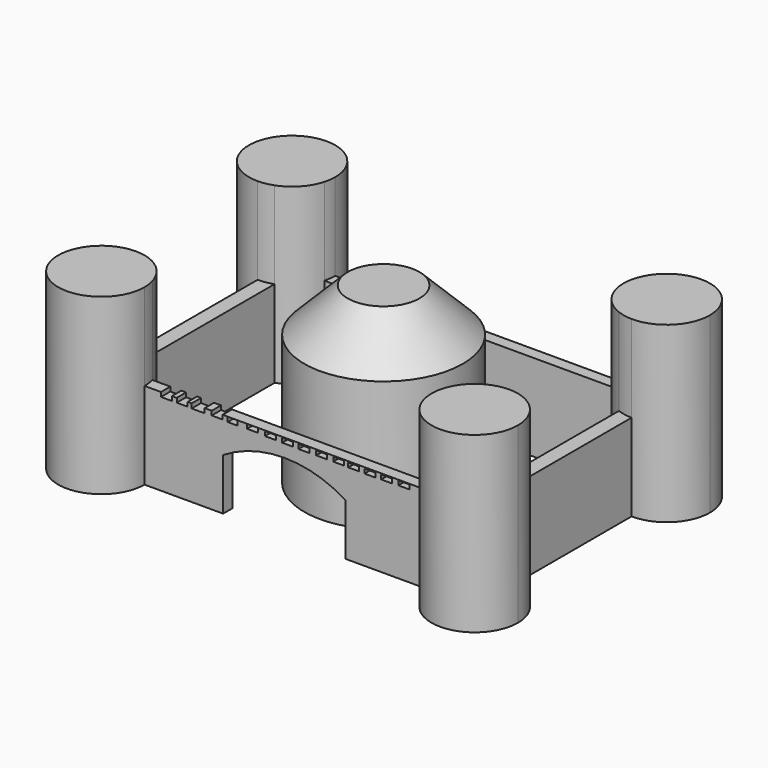
from build123d import *

# Parameters (mm, degrees)
F1_DEPTH   = 25.4
F2_DEPTH   = 50.8
F0_R       = 23.1689364428
F4_DEPTH   = 14.986
F5_W       = 3.2030940056
F5_H       = 1.273414427
F5_H_2     = 1.2491918117
F5_W_2     = 3.7871245295
F5_H_3     = 1.3221087813
F5_H_4     = 1.2197750568
F5_W_3     = 2.9007913545
F5_H_5     = 1.361253047
F1_FACE1_W = 85.1300132265
F1_FACE1_H = 25.4
F1_FACE2_W = 84.1618746061
F1_FACE2_H = 25.4
F6_DEPTH   = 7.112
F7_SIZE    = 12.7


with BuildPart() as f1:
    # F0 (on Top) → F1 (new body)
    with BuildSketch(Plane.XY):
        with BuildLine():
            Line((42.1713891774, 34.8335728049), (-41.9904854287, 34.8335728049))
            ThreePointArc((-41.9904854287, 34.8335728049), (-42.1083213465, 33.1132780775), (-42.4596279258, 31.4251184464))
            Line((-42.4596279258, 31.4251184464), (42.6703853007, 31.4251184464))
            ThreePointArc((42.6703853007, 31.4251184464), (42.3040081413, 33.1122345804), (42.1713891774, 34.8335728049))
        make_face()
    extrude(amount=F1_DEPTH)


with BuildPart() as f1b:
    # F0 (on Top) → F1, piece 2 (new body)
    with BuildSketch(Plane.XY):
        with BuildLine():
            Line((-54.6067543328, 22.2173039008), (-54.6067543328, -22.2160224009))
            ThreePointArc((-54.6067543328, -22.2160224009), (-52.3921133094, -22.4119345582), (-50.2462573349, -22.9935861489))
            Line((-50.2462573349, -22.9935861489), (-50.2462573349, 22.9948099053))
            ThreePointArc((-50.2462573349, 22.9948099053), (-52.3921183776, 22.4132012868), (-54.6067543328, 22.2173039008))
        make_face()
    extrude(amount=F1_DEPTH)


with BuildPart() as f1c:
    # F0 (on Top) → F1, piece 3 (new body)
    with BuildSketch(Plane.XY):
        with BuildLine():
            Line((-41.9913647822, -34.8335728049), (41.9646467417, -34.8335728049))
            ThreePointArc((41.9646467417, -34.8335728049), (42.0972657056, -33.1122345804), (42.463642865, -31.4251184464))
            Line((42.463642865, -31.4251184464), (-42.4599349352, -31.4251184464))
            ThreePointArc((-42.4599349352, -31.4251184464), (-42.1090561661, -33.112226656), (-41.9913645972, -34.8314121366))
            ThreePointArc((-41.9913645972, -34.8314121366), (-41.9913646434, -34.8324924707), (-41.9913647822, -34.8335728049))
        make_face()
    extrude(amount=F1_DEPTH)

    # F3 (on face) → F4 (cut)
    with BuildSketch(Plane.XZ.offset(34.8335728049)):
        with BuildLine():
            Line((-19.0204642713, 15.0923253968), (-19.0204642713, 0))
            Line((-19.0204642713, 0), (16.7462807149, 0))
            Line((16.7462807149, 0), (16.7462807149, 15.0923253968))
            ThreePointArc((16.7462807149, 15.0923253968), (-1.1370917782, 20.2000644219), (-19.0204642713, 15.0923253968))
        make_face()
    extrude(amount=-F4_DEPTH, mode=Mode.SUBTRACT)

    # F5 (on face) + F1_face1 (on face) + F1_face2 (on face) → F6 (cut)
    with BuildSketch(Plane.XZ.offset(34.8335728049)):
        with Locations((-35.5779528618, 24.7632927865)):
            Rectangle(F5_W, F5_H)
        with Locations((-30.9700351208, 24.7754040942)):
            Rectangle(F5_W, F5_H_2)
        with Locations((-26.3112029061, 24.7389456093)):
            Rectangle(F5_W_2, F5_H_3)
        with Locations((-20.7560434937, 24.7901124716)):
            Rectangle(F5_W, F5_H_4)
        with Locations((-16.2332779728, 24.6905572712)):
            Rectangle(F5_W_3, F5_H_5)
        with Locations((-10.4287816212, 24.747133255)):
            Rectangle(F5_W, F5_H)
        with Locations((-5.2050889935, 24.5689451694)):
            Rectangle(F5_W, F5_H)
        with Locations((-0.1880034979, 24.4990028441)):
            Rectangle(F5_W, F5_H)
        with Locations((4.6075105201, 24.4370289147)):
            Rectangle(F5_W, F5_H)
        with Locations((9.7847376019, 24.4842600077)):
            Rectangle(F5_W, F5_H)
        with Locations((14.7634353489, 24.4842600077)):
            Rectangle(F5_W, F5_H)
        with Locations((19.1444754601, 24.4370233268)):
            Rectangle(F5_W, F5_H)
        with Locations((23.9080954343, 24.3755578995)):
            Rectangle(F5_W, F5_H)
        with Locations((28.7535134703, 24.4615059346)):
            Rectangle(F5_W, F5_H)
        with Locations((33.7848700583, 24.5699640363)):
            Rectangle(F5_W, F5_H)
    with BuildSketch(Plane(origin=(0.1053786874, 31.4251184464, 12.7), x_dir=(1, 0, 0), z_dir=(0, -1, 0))):
        Rectangle(F1_FACE1_W, F1_FACE1_H)
    with BuildSketch(Plane(origin=(0.0904518744, 34.8335728049, 12.7), x_dir=(-1, 0, 0), z_dir=(0, 1, 0))):
        Rectangle(F1_FACE2_W, F1_FACE2_H)
    extrude(amount=-F6_DEPTH, dir=(0, -1, 0), mode=Mode.SUBTRACT)


with BuildPart() as f1d:
    # F0 (on Top) → F1, piece 4 (new body)
    with BuildSketch(Plane.XY):
        with BuildLine():
            Line((50.2462573349, 23.1690441136), (50.2462573349, -23.0913582413))
            ThreePointArc((50.2462573349, -23.0913582413), (52.3925594701, -22.5146622382), (54.6067543328, -22.3235281341))
            Line((54.6067543328, -22.3235281341), (54.6067543328, 22.3247913991))
            ThreePointArc((54.6067543328, 22.3247913991), (52.3890618107, 22.553522405), (50.2462573349, 23.1690441136))
        make_face()
    extrude(amount=F1_DEPTH)


with BuildPart() as f2:
    # F0 (on Top) → F2 (new body)
    with BuildSketch(Plane.XY):
        with BuildLine():
            ThreePointArc((-41.9904854287, 34.8335728049), (-63.5278036282, 43.7546221003), (-54.6067543328, 22.2173039008))
            ThreePointArc((-54.6067543328, 22.2173039008), (-52.3921183776, 22.4132012868), (-50.2462573349, 22.9948099053))
            ThreePointArc((-50.2462573349, 22.9948099053), (-45.3389102932, 26.2733562237), (-42.4596279258, 31.4251184464))
            ThreePointArc((-42.4596279258, 31.4251184464), (-42.1083213465, 33.1132780775), (-41.9904854287, 34.8335728049))
        make_face()
    extrude(amount=F2_DEPTH)


with BuildPart() as f2b:
    # F0 (on Top) → F2, piece 2 (new body)
    with BuildSketch(Plane.XY):
        with BuildLine():
            ThreePointArc((42.6703853007, 31.4251184464), (45.4914542286, 26.4098725356), (50.2462573349, 23.1690441136))
            ThreePointArc((50.2462573349, 23.1690441136), (52.3890618107, 22.553522405), (54.6067543328, 22.3247913991))
            ThreePointArc((54.6067543328, 22.3247913991), (63.6442295153, 25.9551457787), (67.4034800242, 34.9397696555))
            ThreePointArc((67.4034800242, 34.9397696555), (54.7341122246, 47.5559268187), (42.1713891774, 34.8335728049))
            ThreePointArc((42.1713891774, 34.8335728049), (42.3040081413, 33.1122345804), (42.6703853007, 31.4251184464))
        make_face()
    extrude(amount=F2_DEPTH)


with BuildPart() as f2c:
    # F0 (on Top) → F2, piece 3 (new body)
    with BuildSketch(Plane.XY):
        with BuildLine():
            ThreePointArc((42.463642865, -31.4251184464), (42.0972657056, -33.1122345804), (41.9646467417, -34.8335728049))
            ThreePointArc((41.9646467417, -34.8335728049), (54.5273697889, -47.5559268187), (67.1967375885, -34.9397696555))
            ThreePointArc((67.1967375885, -34.9397696555), (63.5108065243, -26.0280185859), (54.6067543328, -22.3235281341))
            ThreePointArc((54.6067543328, -22.3235281341), (52.3925594701, -22.5146622382), (50.2462573349, -23.0913582413))
            ThreePointArc((50.2462573349, -23.0913582413), (45.3597287048, -26.3288350204), (42.463642865, -31.4251184464))
        make_face()
    extrude(amount=F2_DEPTH)


with BuildPart() as f2d:
    # F0 (on Top) → F2, piece 4 (new body)
    with BuildSketch(Plane.XY):
        with BuildLine():
            ThreePointArc((-54.6067543328, -22.2160224009), (-63.5279458411, -43.7510758216), (-41.9913647822, -34.8335728049))
            ThreePointArc((-41.9913647822, -34.8335728049), (-41.9913646434, -34.8324924707), (-41.9913645972, -34.8314121366))
            ThreePointArc((-41.9913645972, -34.8314121366), (-42.1090561661, -33.112226656), (-42.4599349352, -31.4251184464))
            ThreePointArc((-42.4599349352, -31.4251184464), (-45.3387686905, -26.2726446835), (-50.2462573349, -22.9935861489))
            ThreePointArc((-50.2462573349, -22.9935861489), (-52.3921133094, -22.4119345582), (-54.6067543328, -22.2160224009))
        make_face()
    extrude(amount=F2_DEPTH)


with BuildPart() as f2e:
    # F0 (on Top) → F2, piece 5 (new body)
    with BuildSketch(Plane.XY):
        Circle(F0_R)
    extrude(amount=F2_DEPTH)

    # F7
    f7_edges = [f2e.edges().sort_by_distance(p)[0] for p in [
        (-23.168936, 0, 50.8),
    ]]
    chamfer(f7_edges, length=F7_SIZE)


solid = Compound([f1.part, f1b.part, f1c.part, f1d.part, f2.part, f2b.part, f2c.part, f2d.part, f2e.part])
